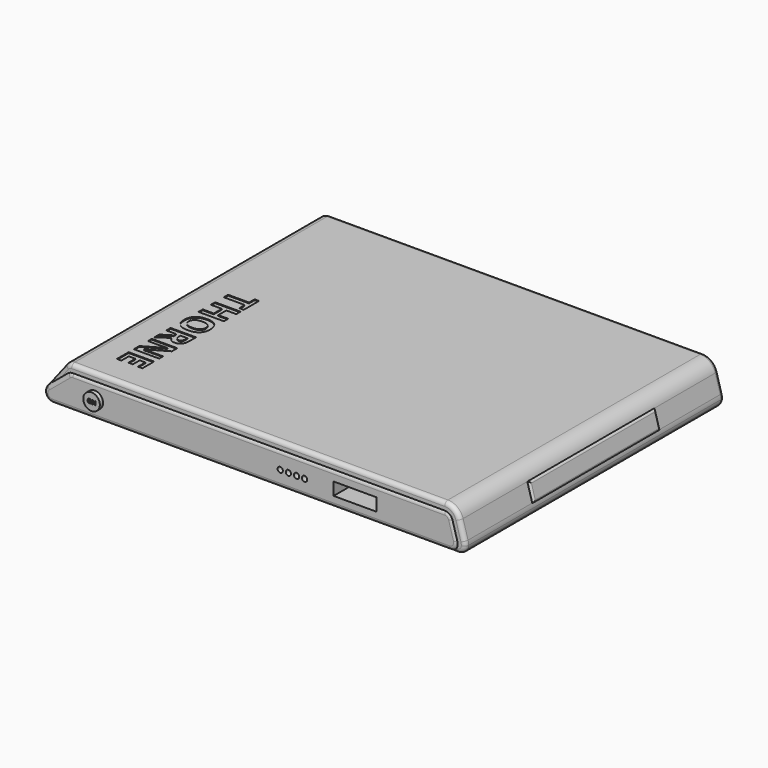
from build123d import *

# Parameters (mm, degrees)
F1_DEPTH      = 80
F2_R          = 0.656282598
F2_W          = 10.6493700296
F2_H          = 3.1434893608
F3_DEPTH      = 10
F4_R          = 2.0498834935
F5_DEPTH      = 1
F6_TEXT_SIZE  = 1.3486456333
F7_DEPTH      = 0.3
F9_DEPTH      = 80
F10_W         = 39.1028262675
F10_H         = 4.4644076265
F11_DEPTH     = 0.5
F12_R         = 0.49999
F13_R         = 1
F14_R         = 1
F15_TEXT_SIZE = 8.8158503382
F16_DEPTH     = 0.2


# Not quite as in the source:
# - a fillet or chamfer is up to 0.001 mm smaller than in the source, because OpenCascade refuses the exact size
# - ends of sketch curves that miss each other by under 0.0002 mm in the source are joined
# - Text() gives the source's letters only with a copy of the font that has no kerning and outlines rounded to 1/6400 em; it was checked with that copy


with BuildPart() as f1:
    # F0 (on Front) → F1 (new body)
    with BuildSketch(Plane.XZ):
        with BuildLine():
            ThreePointArc((-45.5320757336, -29.4630726915), (-46.1322505041, -31.6803658533), (-44.2517072736, -32.9995155334))
            Line((-44.2517072736, -32.9995155334), (54.137341032, -32.9995155334))
            ThreePointArc((54.137341032, -32.9995155334), (55.7323932385, -32.2060844119), (56.0618813839, -30.4553239919))
            Line((56.0618813839, -30.4553239919), (54.8471349496, -26.1593576796))
            ThreePointArc((54.8471349496, -26.1593576796), (54.1291634762, -25.1084970146), (52.9225945977, -24.7035492212))
            Line((52.9225945977, -24.7035492212), (-39.0965453839, -24.7035492212))
            ThreePointArc((-39.0965453839, -24.7035492212), (-39.7773957038, -24.8230059906), (-40.376913844, -25.1671063792))
            add(Edge.make_bspline(
                [(-45.5320757336, -29.4630726915), (-43.8136884371, -28.0310839207), (-42.0953011405, -26.59909515), (-40.376913844, -25.1671063792)],
                knots=[5.524101776, 5.524101776, 5.524101776, 5.524101776, 12.234617454, 12.234617454, 12.234617454, 12.234617454], degree=3))
        make_face()
    extrude(amount=F1_DEPTH)

    # F2 (on face) → F3 (cut)
    with BuildSketch(Plane.XZ.offset(80)):
        with Locations((18.2313658297, -29.0702376515)):
            Circle(F2_R)
        with Locations((12.2167952359, -29.0702376515)):
            Circle(F2_R)
        with Locations((16.258424148, -29.0702376515)):
            Circle(F2_R)
        with Locations((14.2376096919, -29.0702376515)):
            Circle(F2_R)
        with Locations((30.7484706864, -28.8846828043)):
            Rectangle(F2_W, F2_H)
    extrude(amount=-F3_DEPTH, mode=Mode.SUBTRACT)

    # F4 (on face) → F5 (join)
    with BuildSketch(Plane.XZ.offset(80)):
        with Locations((-33.6798354983, -28.7559386343)):
            Circle(F4_R)
    extrude(amount=F5_DEPTH)

    # F6 (on face) → F7 (cut)
    with BuildSketch(Plane.XZ.offset(81)):
        with Locations((-34.7355119884, -29.2543973774)):
            Text('ON', F6_TEXT_SIZE, font='Open Sans', font_style=FontStyle.BOLD, text_align=(TextAlign.LEFT, TextAlign.BOTTOM))
    extrude(amount=-F7_DEPTH, mode=Mode.SUBTRACT)

    # F14
    f14_edges = [f1.edges().sort_by_distance(p)[0] for p in [
        (-44.251707, -40, -32.999516),
        (54.137341, -40, -32.999516),
        (4.942817, 0, -32.999516),
        (4.942817, -80, -32.999516),
    ]]
    fillet(f14_edges, radius=F14_R)


with BuildPart() as f9:
    # F8 (on face) → F9 (new body)
    with BuildSketch(Plane.XZ.offset(80)):
        with BuildLine():
            ThreePointArc((56.061880517, -30.455324237), (55.73239252, -32.2060838684), (54.137341032, -32.9995146325))
            Line((54.137341032, -32.9995146325), (56.0373400767, -32.9995155334))
            ThreePointArc((56.0373400767, -32.9995155334), (57.4515536391, -32.4137290958), (58.0373400767, -30.9995155334))
            ThreePointArc((58.0373400767, -30.9995155334), (58.0003783574, -30.4638522331), (57.8901937989, -29.9383422873))
            Line((57.8901937989, -29.9383422873), (56.6754473647, -25.642375975))
            ThreePointArc((56.6754473647, -25.642375975), (55.2754033344, -23.5931981803), (52.9225945977, -22.8035501765))
            Line((52.9225945977, -22.8035501765), (-39.3971987046, -22.8035501765))
            ThreePointArc((-39.3971987046, -22.8035501765), (-40.2780847191, -23.0079890303), (-40.9788834065, -23.579510347))
            Line((-40.9788834065, -23.579510347), (-45.5320757336, -29.4630726915))
            add(Edge.make_bspline(
                [(-45.5320757336, -29.4630726915), (-43.8136884371, -28.0310839207), (-42.0953011405, -26.59909515), (-40.376913844, -25.1671063792)],
                knots=[0.4262846194, 0.4262846194, 0.4262846194, 0.4262846194, 0.9441225843, 0.9441225843, 0.9441225843, 0.9441225843], degree=3))
            ThreePointArc((-40.376913844, -25.1671063792), (-39.7773953971, -24.8230068377), (-39.0965453839, -24.7035501221))
            Line((-39.0965453839, -24.7035501221), (52.9225945977, -24.7035483203))
            ThreePointArc((52.9225945977, -24.7035483203), (54.1291629327, -25.1084977331), (54.8471340827, -26.1593579247))
            Line((54.8471340827, -26.1593579247), (56.061880517, -30.455324237))
        make_face()
    extrude(amount=-F9_DEPTH)

    # F10 (on face) → F11 (join)
    with BuildSketch(Plane(origin=(45.765483591, 0, 12.9408505474), x_dir=(0, 1, 0), z_dir=(0.9622701759, 0, 0.2720957708))):
        with Locations((-39.5917315036, -42.3282469899)):
            Rectangle(F10_W, F10_H)
    extrude(amount=F11_DEPTH)

    # F12 (radius 0.5 in the source; OpenCascade refuses exactly that, so slightly less here)
    f12_edges = [f9.edges().sort_by_distance(p)[0] for p in [
        (57.156582, -39.591732, -25.506328),
        (57.763956, -59.143145, -27.654311),
        (58.371329, -39.591732, -29.802294),
        (57.763956, -20.040318, -27.654311),
    ]]
    fillet(f12_edges, radius=F12_R)

    # F13
    f13_edges = [f9.edges().sort_by_distance(p)[0] for p in [
        (52.922595, -40, -22.80355),
        (-39.397199, -40, -22.80355),
        (6.762698, -80, -22.80355),
        (6.762698, 0, -22.80355),
    ]]
    fillet(f13_edges, radius=F13_R)

    # F15 (on face) → F16 (cut)
    with BuildSketch(Plane.XY.offset(-22.8035501765)):
        with Locations(Location((-33.8982990648, -36.6017329211), (0, 0, -90))):
            Text('THORNE', F15_TEXT_SIZE, font='Open Sans', font_style=FontStyle.BOLD, text_align=(TextAlign.LEFT, TextAlign.BOTTOM))
    extrude(amount=-F16_DEPTH, mode=Mode.SUBTRACT)


solid = Compound([f1.part, f9.part])
